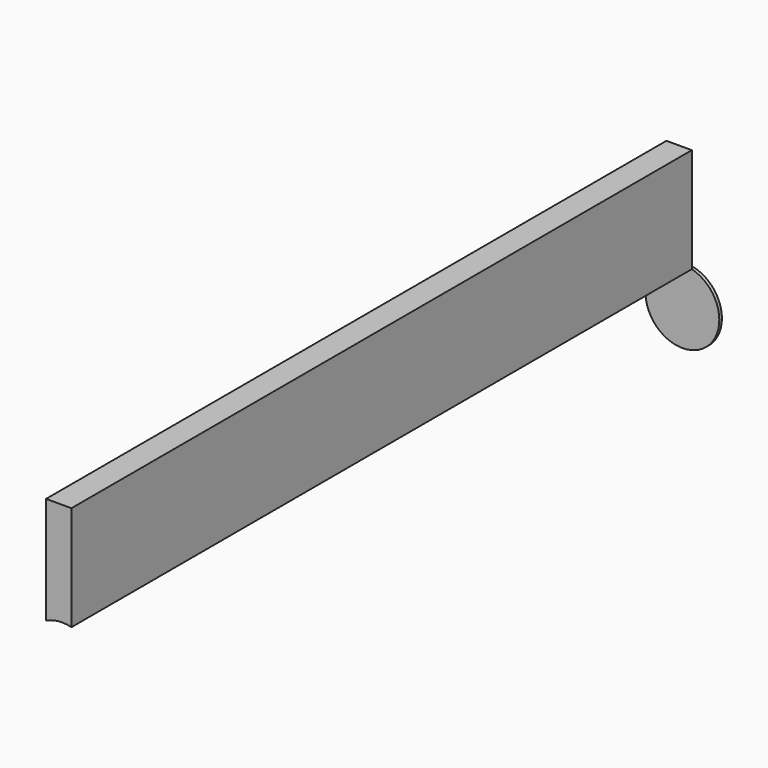
from build123d import *

# Parameters (mm, degrees)
F0_R     = 2.14
F0_R_2   = 0.345
F1_DEPTH = 0.19
F4_DEPTH = 45


# Not quite as in the source:
# - the program builds the solid bodies; features that only make, move or delete a surface that nothing else refers to are left out


with BuildPart() as f1:
    # F0 (on Front) → F1 (new body)
    with BuildSketch(Plane.XZ):
        with Locations((-39.4006967545, 7.7351056971)):
            Circle(F0_R)
        with Locations((-39.4006967545, 7.7351056971)):
            Circle(F0_R_2, mode=Mode.SUBTRACT)
        with Locations((-39.4006967545, 7.7351056971)):
            Circle(F0_R_2)
    extrude(amount=-F1_DEPTH)


with BuildPart() as f4:
    # F3 (on face) → F4 (new body)
    with BuildSketch(Plane.XZ):
        with BuildLine():
            Line((-40.3294656016, 15.8844348318), (-40.3294656016, 9.6630549776))
            ThreePointArc((-40.3294656016, 9.6630549776), (-39.6059801702, 9.8652368478), (-38.8571992517, 9.8049391359))
            Line((-38.8571992517, 9.8049391359), (-38.8571992517, 15.8844348318))
            Line((-38.8571992517, 15.8844348318), (-40.3294656016, 15.8844348318))
        make_face()
    extrude(amount=F4_DEPTH)


solid = Compound([f1.part, f4.part])
